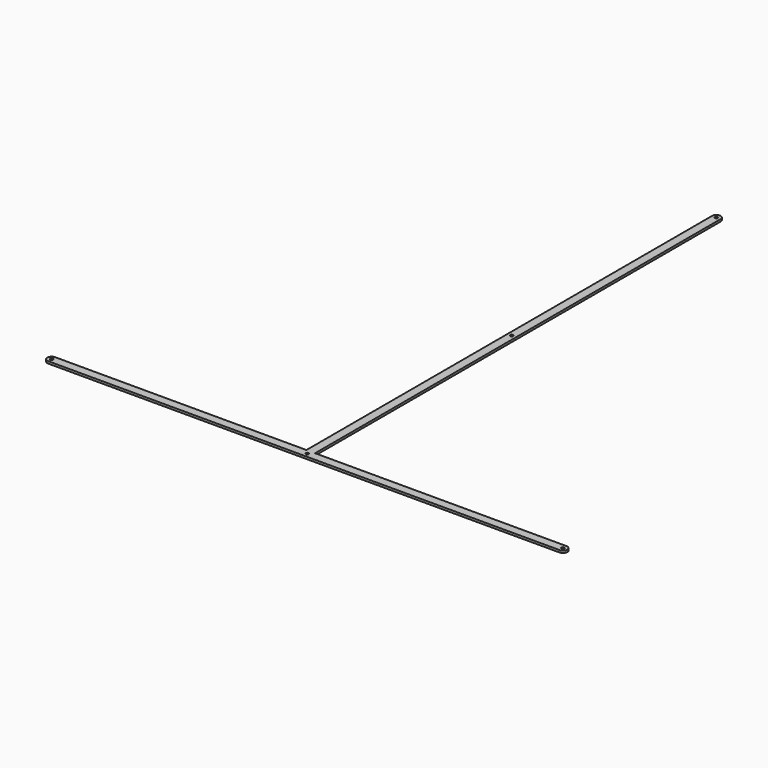
from build123d import *

# Parameters (mm, degrees)
F0_R     = 2.15265
F1_DEPTH = 3.175
F2_R     = 6.34999


# Not quite as in the source:
# - a fillet or chamfer is up to 0.001 mm smaller than in the source, because OpenCascade refuses the exact size


with BuildPart() as f1:
    # F0 (on Top) → F1 (new body)
    with BuildSketch(Plane.XY):
        Polygon((12.7, 749.3), (0, 749.3), (0, 0), (-374.65, 0), (-374.65, -12.7), (387.35, -12.7), (387.35, 0), (12.7, 0), align=None)
        with Locations((-368.3, -6.35)):
            Circle(F0_R, mode=Mode.SUBTRACT)
        with Locations((6.35, -6.35)):
            Circle(F0_R, mode=Mode.SUBTRACT)
        with Locations((381, -6.35)):
            Circle(F0_R, mode=Mode.SUBTRACT)
        with Locations((6.35, 368.3)):
            Circle(F0_R, mode=Mode.SUBTRACT)
        with Locations((6.35, 742.95)):
            Circle(F0_R, mode=Mode.SUBTRACT)
    extrude(amount=F1_DEPTH)

    # F2 (radius 6.35 in the source; OpenCascade refuses exactly that, so slightly less here)
    f2_edges = [f1.edges().sort_by_distance(p)[0] for p in [
        (0, 749.3, 1.5875),
        (12.7, 749.3, 1.5875),
        (387.35, -12.7, 1.5875),
        (387.35, 0, 1.5875),
        (-374.65, -12.7, 1.5875),
        (-374.65, 0, 1.5875),
    ]]
    fillet(f2_edges, radius=F2_R)


solid = f1.part
